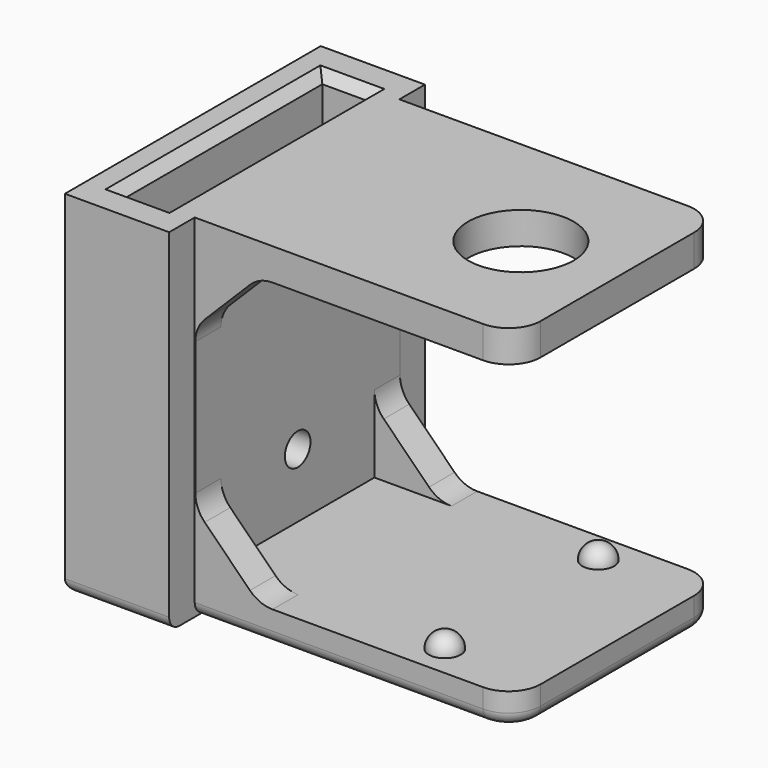
from build123d import *

# Parameters (mm, degrees)
F1_DEPTH  = 40
F2_R      = 8.25
F3_DEPTH  = 5
F4_W      = 5
F4_H      = 55
F4_W_2    = 40
F5_DEPTH  = 16.3
F6_W      = 7
F6_H      = 39
F7_DEPTH  = 55.001
F8_SIZE   = 10
F9_R      = 2.5
F10_DEPTH = 66.401
F11_W     = 30
F11_H     = 10
F12_DEPTH = 50
F13_W     = 30
F13_H     = 10
F14_DEPTH = 50
F15_SIZE  = 1.5
F16_R     = 5
F17_R     = 2.5
F18_DEPTH = 2.5
F19_R     = 2.49999
F20_R     = 2


# Not quite as in the source:
# - a fillet or chamfer is up to 0.001 mm smaller than in the source, because OpenCascade refuses the exact size
# - a feature names something its author has since deleted; it is built from what else it names


with BuildPart() as f1:
    # F0 (on Front) → F1 (new body)
    with BuildSketch(Plane.XZ):
        Polygon((0, 55), (0, 0), (50.1, 0), (50.1, 5), (0.1, 5), (0.1, 50), (50.1, 50), (50.1, 55), align=None)
    extrude(amount=-F1_DEPTH)

    # F2 (on face) → F3 (cut, through all)
    with BuildSketch(Plane.XY.offset(55)):
        with Locations((35, 20)):
            Circle(F2_R)
    extrude(amount=-F3_DEPTH, mode=Mode.SUBTRACT)

    # F4 (on face) → F5 (join)
    with BuildSketch(Plane(origin=(0, 0, 0), x_dir=(0, -1, 0), z_dir=(-1, 0, 0))):
        with Locations((2.5, 27.5)):
            Rectangle(F4_W, F4_H)
        with Locations((-20, 27.5)):
            Rectangle(F4_W_2, F4_H)
        with Locations((-42.5, 27.5)):
            Rectangle(F4_W, F4_H)
    extrude(amount=F5_DEPTH)

    # F6 (on face) → F7 (cut, through all)
    with BuildSketch(Plane(origin=(0, 0, 0), x_dir=(1, 0, 0), z_dir=(0, 0, -1))):
        with Locations((-8.15, -20)):
            Rectangle(F6_W, F6_H)
    extrude(amount=-F7_DEPTH, mode=Mode.SUBTRACT)

    # F8
    f8_edges = [f1.edges().sort_by_distance(p)[0] for p in [
        (0.1, 20, 5),
        (0.1, 20, 50),
    ]]
    chamfer(f8_edges, length=F8_SIZE)

    # F9 (on face) → F10 (cut, through all)
    with BuildSketch(Plane(origin=(-16.3, 0, 0), x_dir=(0, -1, 0), z_dir=(-1, 0, 0))):
        with Locations((-20, 15)):
            Circle(F9_R)
        with Locations((-20, 40)):
            Circle(F9_R)
    extrude(amount=-F10_DEPTH, mode=Mode.SUBTRACT)

    # F11 (on face) → F12 (cut)
    with BuildSketch(Plane.YZ.offset(50.1)):
        with Locations((20, 10)):
            Rectangle(F11_W, F11_H)
    extrude(amount=-F12_DEPTH, mode=Mode.SUBTRACT)

    # F13 (on face) → F14 (cut)
    with BuildSketch(Plane.YZ.offset(50.1)):
        with Locations((20, 45)):
            Rectangle(F13_W, F13_H)
    extrude(amount=-F14_DEPTH, mode=Mode.SUBTRACT)

    # F15
    f15_edges = [f1.edges().sort_by_distance(p)[0] for p in [
        (-11.65, 20, 55),
        (-8.15, 39.5, 55),
        (-4.65, 20, 55),
        (-8.15, 0.5, 55),
        (-11.65, 20, 0),
        (-8.15, 0.5, 0),
        (-4.65, 20, 0),
        (-8.15, 39.5, 0),
    ]]
    chamfer(f15_edges, length=F15_SIZE)

    # F16
    f16_edges = [f1.edges().sort_by_distance(p)[0] for p in [
        (50.1, 0, 52.5),
        (50.1, 40, 52.5),
        (50.1, 40, 2.5),
        (50.1, 0, 2.5),
        (0.1, 37.5, 15),
        (0.1, 2.5, 15),
        (10.1, 2.5, 5),
        (10.1, 37.5, 5),
        (0.1, 2.5, 40),
        (0.1, 37.5, 40),
        (10.1, 37.5, 50),
        (10.1, 2.5, 50),
    ]]
    fillet(f16_edges, radius=F16_R)

    # F17 (on face) → F18 (join)
    with BuildSketch(Plane.XY.offset(5)):
        with Locations((35.1, 5)):
            Circle(F17_R)
        with Locations((35.1, 35)):
            Circle(F17_R)
    extrude(amount=F18_DEPTH)

    # F19 (radius 2.5 in the source; OpenCascade refuses exactly that, so slightly less here)
    f19_edges = [f1.edges().sort_by_distance(p)[0] for p in [
        (32.6, 5, 7.5),
        (32.6, 35, 7.5),
    ]]
    fillet(f19_edges, radius=F19_R)

    # F20
    f20_edges = [f1.edges().sort_by_distance(p)[0] for p in [
        (-8.15, -5, 0),
        (-8.15, 45, 0),
        (-16.3, 20, 0),
        (22.55, 40, 0),
    ]]
    fillet(f20_edges, radius=F20_R)


solid = f1.part
